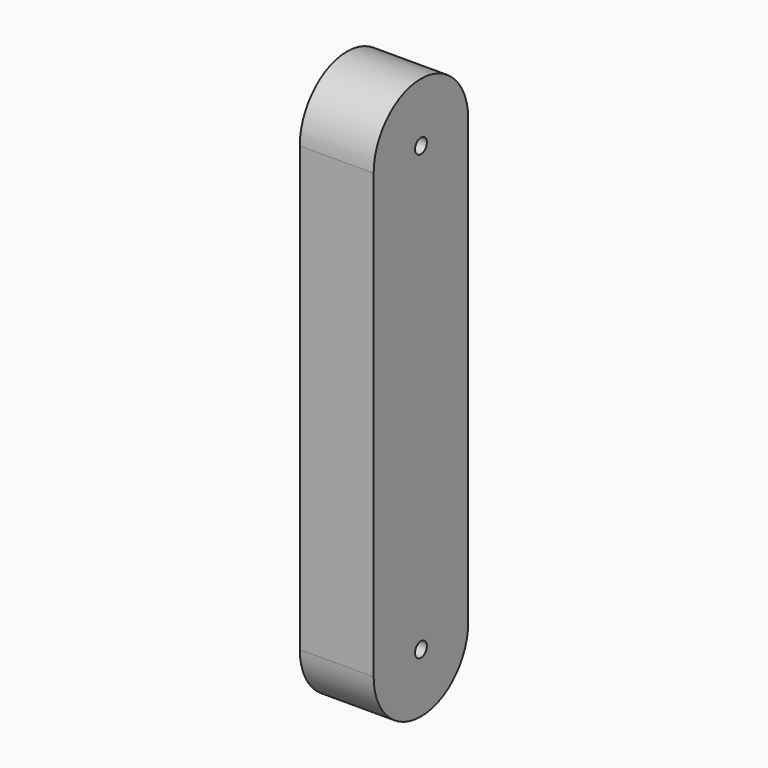
from build123d import *

# Parameters (mm, degrees)
F0_R     = 2.5
F1_DEPTH = 25


# Not quite as in the source:
# - the program builds the solid bodies; features that only make, move or delete a surface that nothing else refers to are left out


with BuildPart() as f1:
    # F0 (on Right) → F1 (new body)
    with BuildSketch(Plane.YZ):
        with BuildLine():
            Line((0, 150), (0, 0))
            ThreePointArc((0, 0), (20, -20), (40, 0))
            Line((40, 0), (40, 150))
            ThreePointArc((40, 150), (20, 170), (0, 150))
        make_face()
        with Locations((20, 0)):
            Circle(F0_R, mode=Mode.SUBTRACT)
        with Locations((20, 150)):
            Circle(F0_R, mode=Mode.SUBTRACT)
    extrude(amount=F1_DEPTH)


solid = f1.part
